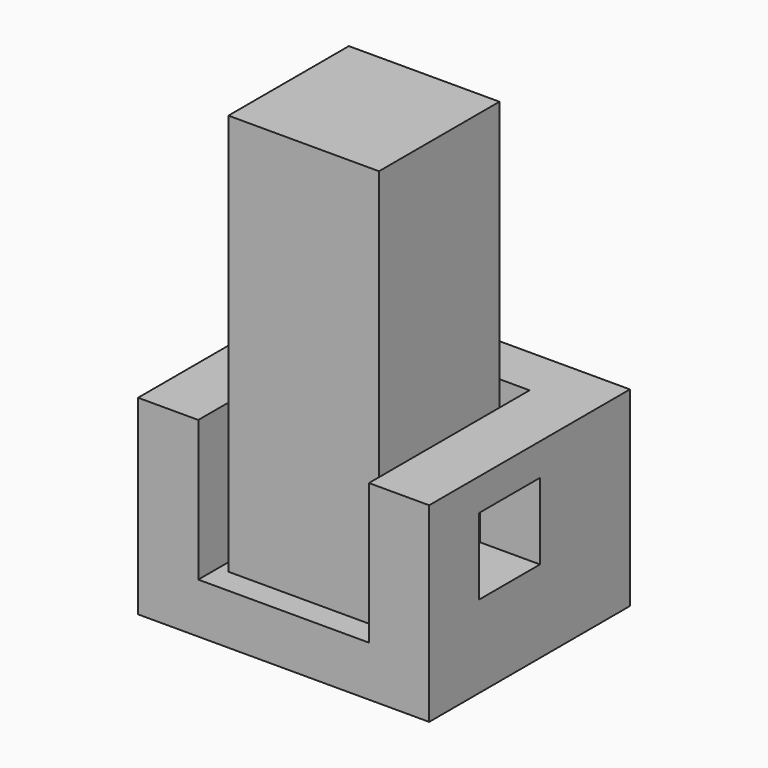
from build123d import *

# Parameters (mm, degrees)
F0_W     = 15
F0_H     = 15
F1_DEPTH = 40
F3_DEPTH = 14
F5_W     = 7.6
F5_H     = 7.6
F6_DEPTH = 20
F2_W     = 17
F2_H     = 20
F7_DEPTH = 5


with BuildPart() as f1:
    # F0 (on Top) → F1 (new body)
    with BuildSketch(Plane.XY):
        with Locations((7.5, 10)):
            Rectangle(F0_W, F0_H)
    extrude(amount=F1_DEPTH)


with BuildPart() as f3:
    # F2 (on Top) → F3 (new body)
    with BuildSketch(Plane.XY):
        Polygon((-7, 0), (-1, 0), (-1, 20), (16, 20), (16, 0), (22, 0), (22, 25), (-7, 25), align=None)
    extrude(amount=F3_DEPTH)

    # F5 (on offset) → F6 (cut)
    with BuildSketch(Plane.YZ.offset(22)):
        with Locations((10, 7)):
            Rectangle(F5_W, F5_H)
    extrude(amount=-F6_DEPTH, mode=Mode.SUBTRACT)

    # F2 (on Top) → F7 (join)
    with BuildSketch(Plane.XY):
        Polygon((-7, 0), (-1, 0), (-1, 20), (16, 20), (16, 0), (22, 0), (22, 25), (-7, 25), align=None)
        with Locations((7.5, 10)):
            Rectangle(F2_W, F2_H)
    extrude(amount=-F7_DEPTH)


solid = Compound([f1.part, f3.part])
